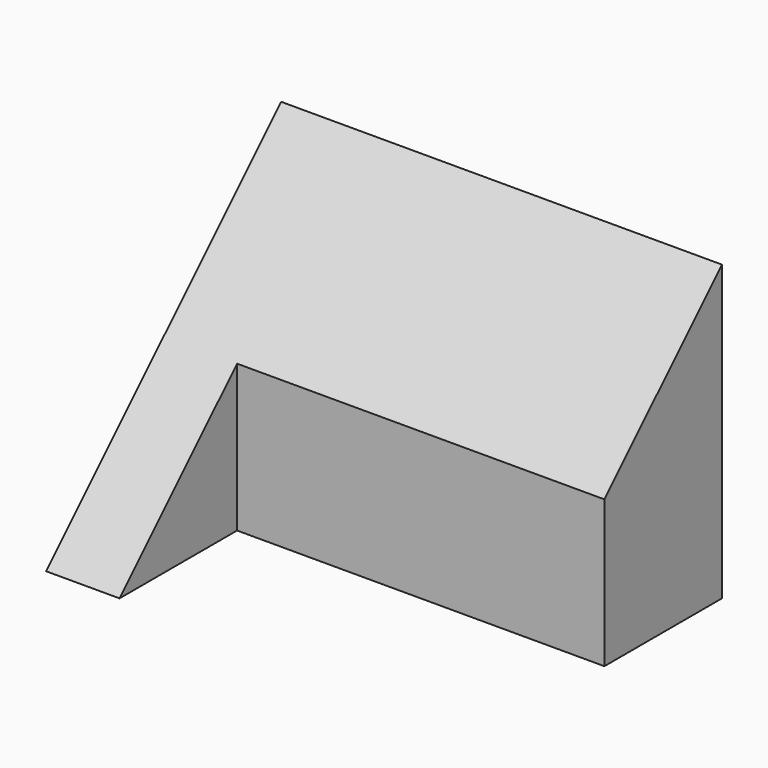
from build123d import *

# Parameters (mm, degrees)
F1_DEPTH = 38.1
F3_DEPTH = 6.35


# Not quite as in the source:
# - the program builds the solid bodies; features that only make, move or delete a surface that nothing else refers to are left out


with BuildPart() as f1:
    # F0 (on Right) → F1 (new body)
    with BuildSketch(Plane.YZ):
        Polygon((12.7, 0), (25.4, 0), (25.4, 25.4), (12.7, 12.7), align=None)
    extrude(amount=F1_DEPTH)

    # F2 (on Right) → F3 (join)
    with BuildSketch(Plane.YZ):
        Polygon((12.7, 12.7), (0, 0), (12.7, 0), align=None)
    extrude(amount=F3_DEPTH)


solid = f1.part
